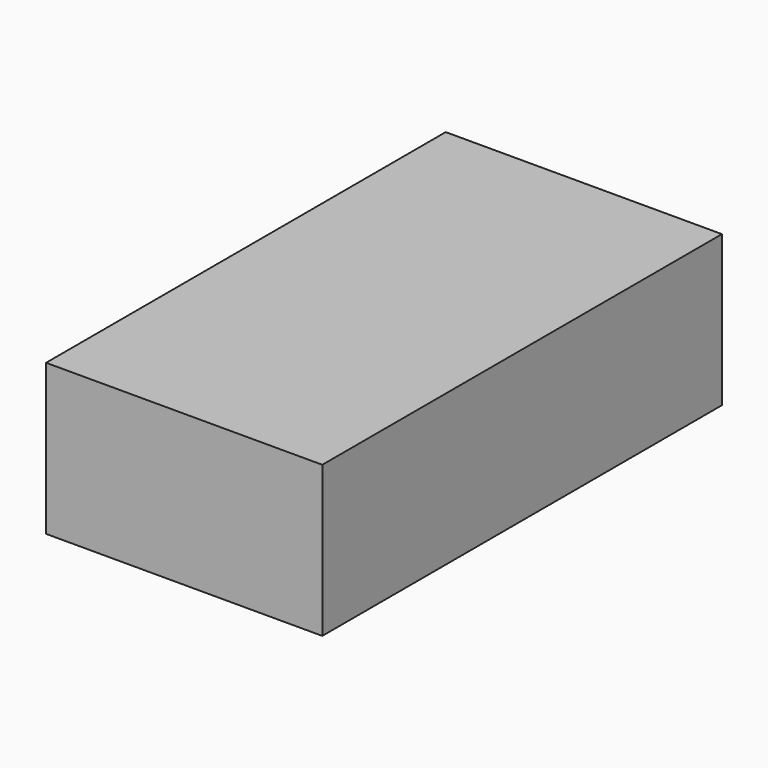
from build123d import *

# Parameters (mm, degrees)
F0_W     = 55
F0_H     = 30
F1_DEPTH = 30
F2_DEPTH = 69.4722199


# Not quite as in the source:
# - an extrude ends at something that could not be found from the text; its depth is read off the source's solid


with BuildPart() as f1:
    # F0 (on Front) → F1 (new body)
    with BuildSketch(Plane.XZ):
        Rectangle(F0_W, F0_H)
    extrude(amount=F1_DEPTH)

    # F2 (add, through all): a face of the model
    f2_faces = [f1.faces().sort_by_distance(p)[0] for p in [
        (0, -30, 0),
    ]]
    extrude(f2_faces, amount=F2_DEPTH)


solid = f1.part
